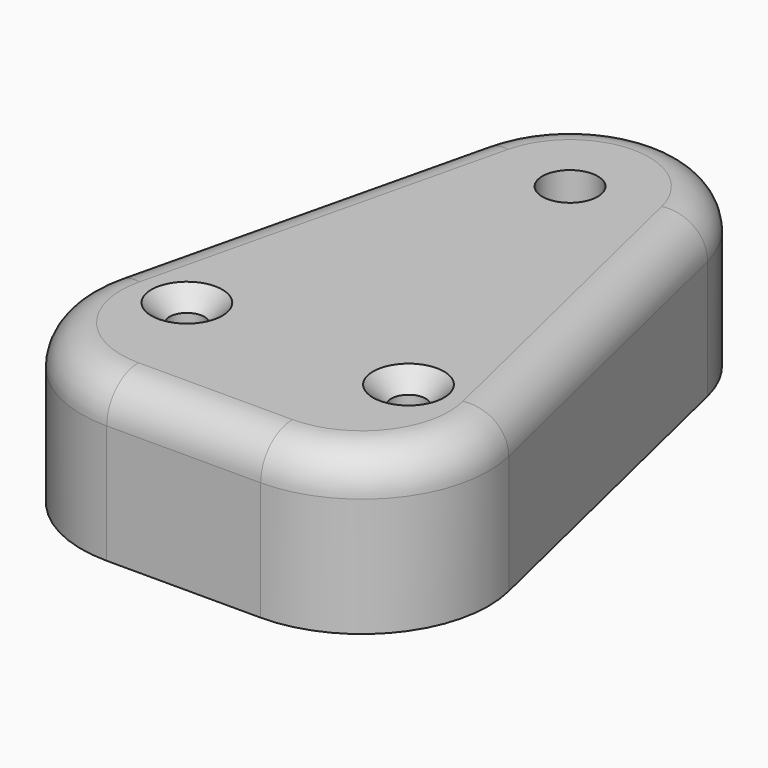
from build123d import *

# Parameters (mm, degrees)
F1_DEPTH       = 20
F2_D           = 4.4
F2_CSINK_D     = 8.96
F2_CSINK_ANGLE = 90
F3_R           = 5
F4_D           = 7


# Not quite as in the source:
# - a feature names something its author has since deleted; it is built from what else it names


with BuildPart() as f1:
    # F0 (on Top) → F1 (new body)
    with BuildSketch(Plane.XY):
        with BuildLine():
            Line((-9.7258236175, -61), (9.7258236175, -61))
            ThreePointArc((9.7258236175, -61), (22.2857339512, -54.9120458236), (25.2876244635, -41.2810815511))
            Line((25.2876244635, -41.2810815511), (14.5891882931, 3.4864860458))
            ThreePointArc((14.5891882931, 3.4864860458), (0, 15), (-14.5891882931, 3.4864860458))
            Line((-14.5891882931, 3.4864860458), (-25.2876244635, -41.2810815511))
            ThreePointArc((-25.2876244635, -41.2810815511), (-22.2857339512, -54.9120458236), (-9.7258236175, -61))
        make_face()
    extrude(amount=-F1_DEPTH)

    # F2 (through all)
    with Locations(Plane.XY):
        with Locations((-14, -43), (14, -43)):
            CounterSinkHole(F2_D / 2, F2_CSINK_D / 2, counter_sink_angle=F2_CSINK_ANGLE)

    # F3
    f3_edges = [f1.edges().sort_by_distance(p)[0] for p in [
        (0, -61, 0),
        (-19.938406, -18.897298, 0),
        (19.938406, -18.897298, 0),
    ]]
    fillet(f3_edges, radius=F3_R)

    # F4 (through all)
    with Locations(Plane.XY):
        with Locations((0, 0)):
            Hole(F4_D / 2)


solid = f1.part
